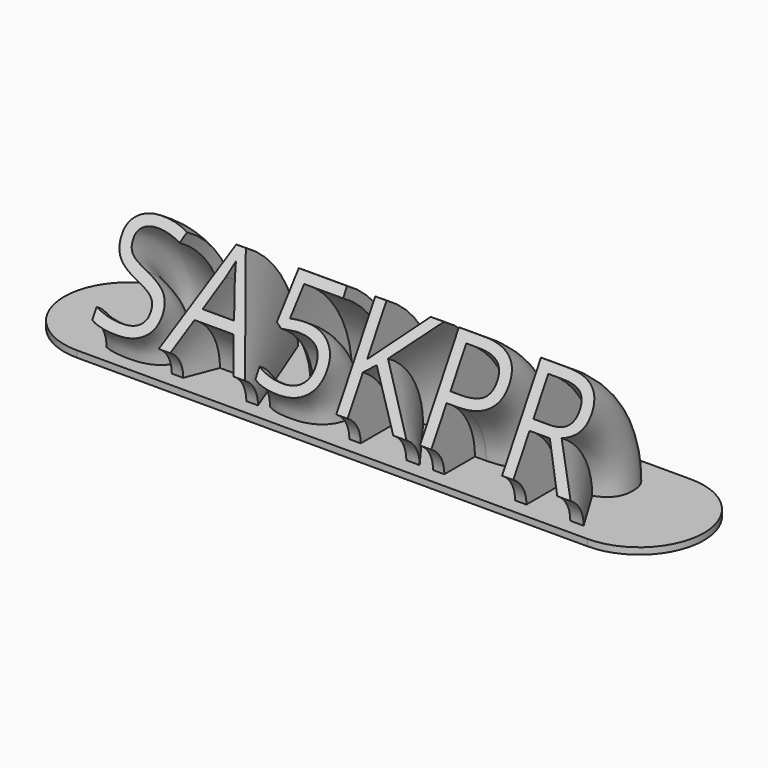
from build123d import *

# Parameters (mm, degrees)
F0_TEXT_SIZE = 41.6666666667
F1_ANGLE     = 60
F3_DEPTH     = 2


# Not quite as in the source:
# - Text() gives the source's letters only with a copy of the font that has no kerning and outlines rounded to 1/6400 em; it was checked with that copy


with BuildPart() as f1:
    # F0 (on Top) → F1 (revolve)
    with BuildSketch(Plane.XY):
        with Locations((-75.732421875, -15)):
            Text('SA5KPR', F0_TEXT_SIZE, font='Open Sans', text_align=(TextAlign.LEFT, TextAlign.BOTTOM))
    revolve(axis=Axis((0, -25, 0), (1, 0, 0)), revolution_arc=F1_ANGLE)

    # F2 (on Top) → F3 (join)
    with BuildSketch(Plane.XY):
        with BuildLine():
            ThreePointArc((-78.0305989583, 19.74609375), (-97.7766927083, 0), (-78.0305989583, -19.74609375))
            Line((-78.0305989583, -19.74609375), (78.0305989583, -19.74609375))
            ThreePointArc((78.0305989583, -19.74609375), (97.7766927083, 0), (78.0305989583, 19.74609375))
            Line((78.0305989583, 19.74609375), (-78.0305989583, 19.74609375))
        make_face()
    extrude(amount=-F3_DEPTH)


solid = f1.part
